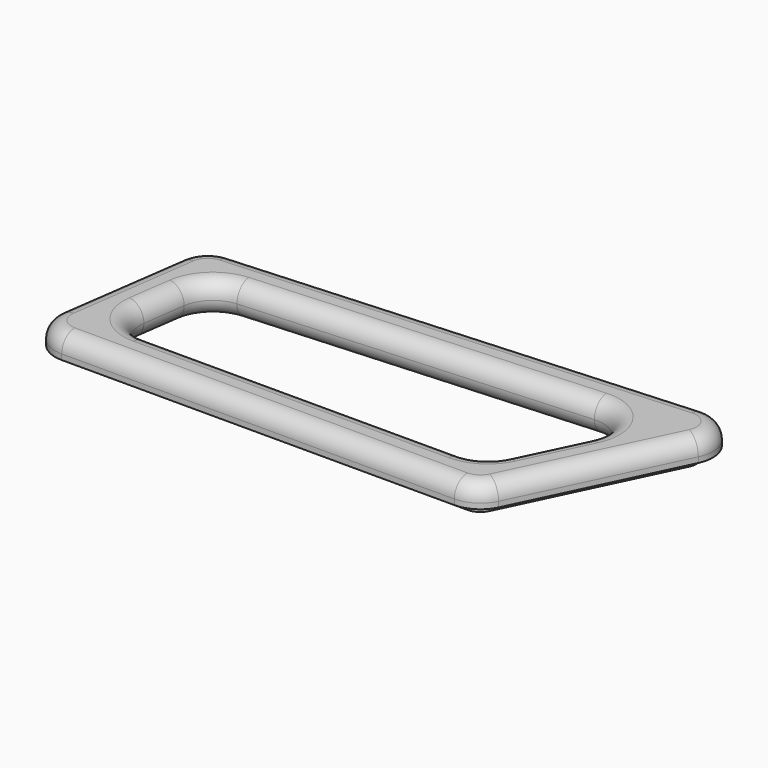
from build123d import *

# Parameters (mm, degrees)
F1_DEPTH = 3
F2_R     = 1.49999
F5_DEPTH = 1


# Not quite as in the source:
# - a fillet or chamfer is up to 0.001 mm smaller than in the source, because OpenCascade refuses the exact size
# - a feature names something its author has since deleted; it is built from what else it names


with BuildPart() as f1:
    # F0 (on Top) → F1 (new body)
    with BuildSketch(Plane.XY):
        with BuildLine():
            ThreePointArc((7.7126204308, 17.4904861667), (5.8623387123, 16.6961416403), (4.9310753592, 14.9108477622))
            Line((4.9310753592, 14.9108477622), (3.2946010031, 3.1761362209))
            ThreePointArc((3.2946010031, 3.1761362209), (4.002766576, 0.7923969722), (6.265847815, -0.2382215753))
            Line((6.265847815, -0.2382215753), (42.381050937, -0.2382215753))
            ThreePointArc((42.381050937, -0.2382215753), (43.9792635765, 0.2229368859), (45.0861233616, 1.4646341854))
            Line((45.0861233616, 1.4646341854), (51.9699000588, 15.820103651))
            ThreePointArc((51.9699000588, 15.820103651), (51.7518427103, 18.7949713512), (49.0751258939, 20.1112440911))
            Line((49.0751258939, 20.1112440911), (7.7126204308, 17.4904861667))
        make_face()
        with BuildLine():
            Line((39.8630322028, 3.7617784247), (10.8623798602, 3.7617784247))
            ThreePointArc((10.8623798602, 3.7617784247), (8.5992986212, 4.7923969722), (7.8911330484, 7.1761362209))
            Line((7.8911330484, 7.1761362209), (8.4418632915, 11.125272678))
            ThreePointArc((8.4418632915, 11.125272678), (9.3731266446, 12.9105665561), (11.2234083631, 13.7049110825))
            Line((11.2234083631, 13.7049110825), (42.5178482436, 15.6877491719))
            ThreePointArc((42.5178482436, 15.6877491719), (45.19456506, 14.3714764321), (45.4126224085, 11.3966087319))
            Line((45.4126224085, 11.3966087319), (42.5681046274, 5.4646341854))
            ThreePointArc((42.5681046274, 5.4646341854), (41.4612448422, 4.2229368859), (39.8630322028, 3.7617784247))
        make_face(mode=Mode.SUBTRACT)
    extrude(amount=-F1_DEPTH)

    # F2 (radius 1.5 in the source; OpenCascade refuses exactly that, so slightly less here)
    f2_edges = [f1.edges().sort_by_distance(p)[0] for p in [
        (24.323449, -0.238222, 0),
        (48.528012, 8.642369, 0),
        (28.393873, 18.800865, 0),
        (4.112838, 9.043492, 0),
        (25.362706, 3.761778, 0),
        (8.166498, 9.150704, 0),
        (43.990364, 8.430621, 0),
        (26.870628, 14.69633, 0),
        (8.166498, 9.150704, -3),
        (25.362706, 3.761778, -3),
        (26.870628, 14.69633, -3),
        (43.990364, 8.430621, -3),
    ]]
    fillet(f2_edges, radius=F2_R)

    # F4 (on offset) → F5 (cut)
    with BuildSketch(Plane(origin=(0, 0, -3), x_dir=(1, 0, 0), z_dir=(0, 0, -1))):
        with BuildLine():
            Line((3.2946010031, -3.1761362209), (4.9310753592, -14.9108477622))
            ThreePointArc((4.9310753592, -14.9108477622), (5.8623387123, -16.6961416403), (7.7126204308, -17.4904861667))
            Line((7.7126204308, -17.4904861667), (49.0751258939, -20.1112440911))
            ThreePointArc((49.0751258939, -20.1112440911), (51.7518427103, -18.7949713512), (51.9699000588, -15.820103651))
            Line((51.9699000588, -15.820103651), (45.0861233616, -1.4646341854))
            ThreePointArc((45.0861233616, -1.4646341854), (43.9792635765, -0.2229368859), (42.381050937, 0.2382215753))
            Line((42.381050937, 0.2382215753), (6.265847815, 0.2382215753))
            ThreePointArc((6.265847815, 0.2382215753), (4.002766576, -0.7923969722), (3.2946010031, -3.1761362209))
        make_face()
        with BuildLine():
            ThreePointArc((50.6173638465, -16.4686757707), (50.5083351723, -17.9561096208), (49.1699767641, -18.6142459907))
            Line((49.1699767641, -18.6142459907), (7.8074713009, -15.9934880663))
            ThreePointArc((7.8074713009, -15.9934880663), (6.8823304417, -15.5963158031), (6.4166987651, -14.7036688641))
            Line((6.4166987651, -14.7036688641), (4.7802244091, -2.9689573228))
            ThreePointArc((4.7802244091, -2.9689573228), (5.1343071955, -1.7770876984), (6.265847815, -1.2617784247))
            Line((6.265847815, -1.2617784247), (42.381050937, -1.2617784247))
            ThreePointArc((42.381050937, -1.2617784247), (43.1801572567, -1.4923576553), (43.7335871493, -2.113206305))
            Line((43.7335871493, -2.113206305), (50.6173638465, -16.4686757707))
        make_face(mode=Mode.SUBTRACT)
    extrude(amount=-F5_DEPTH, mode=Mode.SUBTRACT)


solid = f1.part
